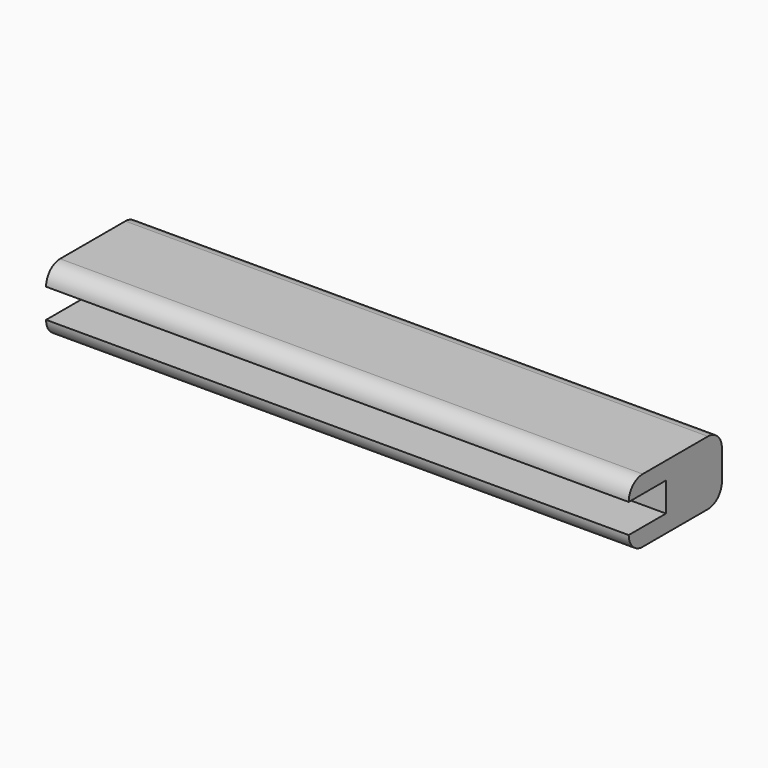
from build123d import *

# Parameters (mm, degrees)
F0_W     = 100
F0_H     = 11
F1_DEPTH = 20
F2_W     = 100
F2_H     = 5
F3_DEPTH = 8
F4_R     = 2.99999


# Not quite as in the source:
# - a fillet or chamfer is up to 0.001 mm smaller than in the source, because OpenCascade refuses the exact size


with BuildPart() as f1:
    # F0 (on Front) → F1 (new body)
    with BuildSketch(Plane.XZ):
        Rectangle(F0_W, F0_H)
    extrude(amount=-F1_DEPTH)

    # F2 (on face) → F3 (cut)
    with BuildSketch(Plane.XZ):
        Rectangle(F2_W, F2_H)
    extrude(amount=-F3_DEPTH, mode=Mode.SUBTRACT)

    # F4 (radius 3 in the source; OpenCascade refuses exactly that, so slightly less here)
    f4_edges = [f1.edges().sort_by_distance(p)[0] for p in [
        (0, 20, 5.5),
        (0, 20, -5.5),
        (0, 0, 5.5),
        (0, 0, -5.5),
    ]]
    fillet(f4_edges, radius=F4_R)


solid = f1.part
